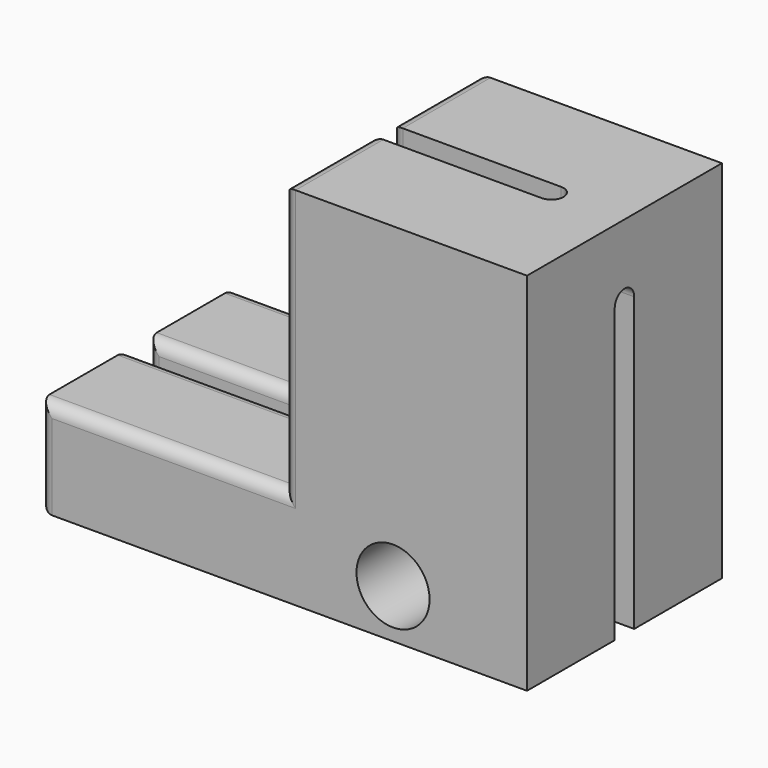
from build123d import *

# Parameters (mm, degrees)
F0_R     = 15
F1_DEPTH = 100
F3_DEPTH = 150
F5_R     = 5
F7_DEPTH = 300


# Not quite as in the source:
# - the program builds the solid bodies; features that only make, move or delete a surface that nothing else refers to are left out


with BuildPart() as f1:
    # F0 (on Front) → F1 (new body)
    with BuildSketch(Plane.XZ):
        Polygon((0, 40), (0, 0), (200, 0), (200, 150), (100, 150), (100, 40), align=None)
        with Locations((145, 20)):
            Circle(F0_R, mode=Mode.SUBTRACT)
    extrude(amount=F1_DEPTH)

    # F2 (on Top) → F3 (cut, through all)
    with BuildSketch(Plane.XY):
        with BuildLine():
            Line((-30, -55), (170, -55))
            ThreePointArc((170, -55), (175, -50), (170, -45))
            Line((170, -45), (-30, -45))
            Line((-30, -45), (-30, -55))
        make_face()
    extrude(amount=F3_DEPTH, mode=Mode.SUBTRACT)

    # F5
    f5_edges = [f1.edges().sort_by_distance(p)[0] for p in [
        (100, -45, 95),
        (100, -55, 95),
        (100, -100, 95),
        (50, -100, 40),
        (50, -55, 40),
        (50, -45, 40),
        (100, 0, 95),
        (50, 0, 40),
        (0, 0, 20),
        (0, -45, 20),
        (0, -22.5, 0),
        (0, -55, 20),
        (0, -100, 20),
        (0, -77.5, 0),
        (100, -22.5, 150),
        (100, -77.5, 150),
    ]]
    fillet(f5_edges, radius=F5_R)

    # F6 (on face) → F7 (cut)
    with BuildSketch(Plane.YZ.offset(200)):
        with BuildLine():
            Line((-45, -10), (-45, 120))
            ThreePointArc((-45, 120), (-50, 125), (-55, 120))
            Line((-55, 120), (-55, -10))
            Line((-55, -10), (-45, -10))
        make_face()
    extrude(amount=-F7_DEPTH, mode=Mode.SUBTRACT)


solid = f1.part
